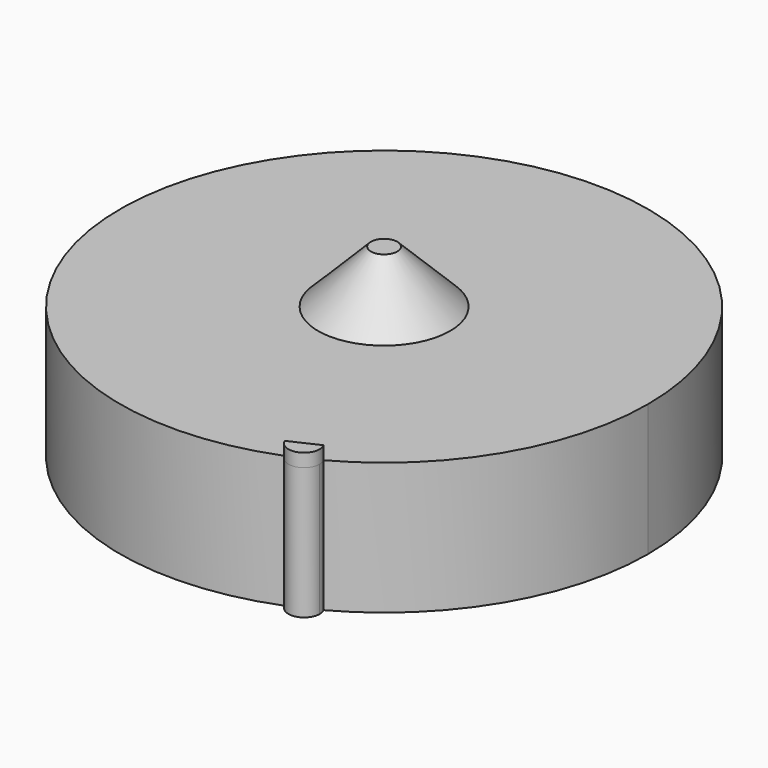
from build123d import *

# Parameters (mm, degrees)
F0_R     = 6.35
F1_DEPTH = 12.7
F2_DEPTH = 17.78
F3_SIZE  = 5.07999
F5_DEPTH = 1.27


# Not quite as in the source:
# - a fillet or chamfer is up to 0.001 mm smaller than in the source, because OpenCascade refuses the exact size


with BuildPart() as f1:
    # F0 (on Top) → F1 (new body)
    with BuildSketch(Plane.XY):
        with BuildLine():
            ThreePointArc((12.068946544, -22.3495084805), (21.8141151805, -13.011701614), (25.4, 0))
            ThreePointArc((25.4, 0), (-21.0057565892, 14.2799926511), (9.3434495971, -23.6190590335))
            ThreePointArc((9.3434495971, -23.6190590335), (10.0899459577, -21.6613011879), (12.068946544, -22.3495084805))
        make_face()
        Circle(F0_R, mode=Mode.SUBTRACT)
        with BuildLine():
            ThreePointArc((12.068946544, -22.3495084805), (10.0899459577, -21.6613011879), (9.3434495971, -23.6190590335))
            ThreePointArc((9.3434495971, -23.6190590335), (10.7249996167, -23.0246472986), (12.068946544, -22.3495084805))
        make_face()
        with BuildLine():
            ThreePointArc((12.068946544, -22.3495084805), (10.7249996167, -23.0246472986), (9.3434495971, -23.6190590335))
            ThreePointArc((9.3434495971, -23.6190590335), (11.0284458537, -24.4977142177), (12.2289962148, -23.0246472986))
            ThreePointArc((12.2289962148, -23.0246472986), (12.1884369016, -22.677722119), (12.068946544, -22.3495084805))
        make_face()
    extrude(amount=F1_DEPTH)

    # F0 (on Top) → F2 (join)
    with BuildSketch(Plane.XY):
        Circle(F0_R)
    extrude(amount=F2_DEPTH)

    # F3 (size 5.08 in the source; OpenCascade refuses exactly that, so slightly less here)
    f3_edges = [f1.edges().sort_by_distance(p)[0] for p in [
        (-6.35, 0, 17.78),
    ]]
    chamfer(f3_edges, length=F3_SIZE)

    # F4 (on face) → F5 (join)
    with BuildSketch(Plane.XY.offset(12.7)):
        with BuildLine():
            Line((12.068946544, -22.3495084805), (9.3434495971, -23.6190590335))
            ThreePointArc((9.3434495971, -23.6190590335), (11.3711055832, -24.4117207278), (12.068946544, -22.3495084805))
        make_face()
    extrude(amount=F5_DEPTH)


solid = f1.part
